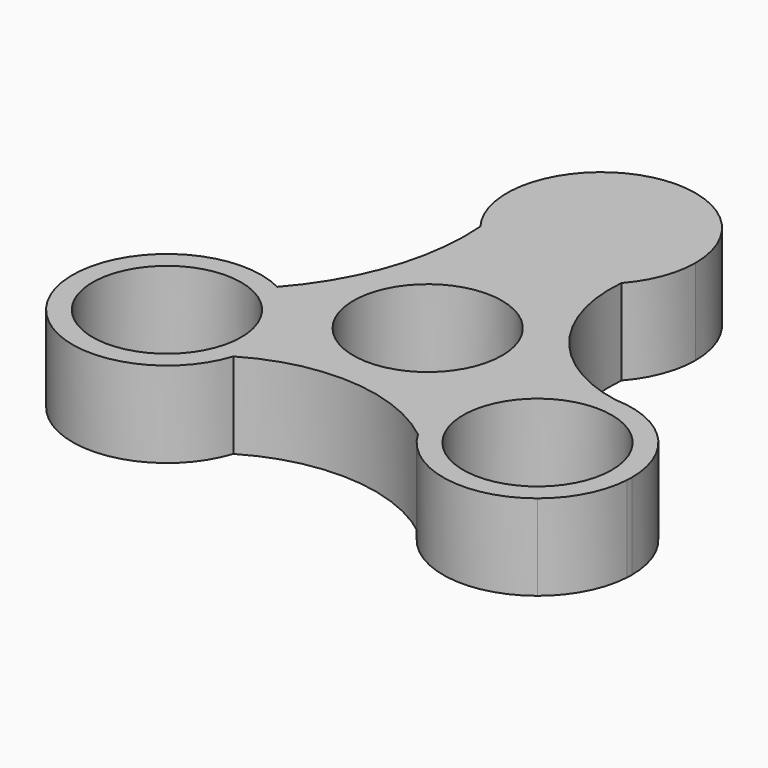
from build123d import *

# Parameters (mm, degrees)
F0_R     = 10.9982
F0_R_2   = 13.97
F1_DEPTH = 12.7


with BuildPart() as f1:
    # F0 (on Top) → F1 (new body)
    with BuildSketch(Plane.XY):
        with BuildLine():
            ThreePointArc((13.97, 32.0970378816), (12.2885629968, 38.7417440057), (7.6490093808, 43.7869290484))
            ThreePointArc((7.6490093808, 43.7869290484), (0, 44.45), (-7.6490093808, 43.7869290484))
            ThreePointArc((-7.6490093808, 43.7869290484), (-13.7655856932, 34.4781196782), (-11.1311920138, 23.6556242351))
            ThreePointArc((-11.1311920138, 23.6556242351), (-0.5487801971, 18.1378208443), (10.4341459432, 22.8078237902))
            ThreePointArc((10.4341459432, 22.8078237902), (13.0561464228, 27.1273356182), (13.97, 32.0970378816))
        make_face()
        with Locations((0, 32.0970378816)):
            Circle(F0_R, mode=Mode.SUBTRACT)
        with BuildLine():
            ThreePointArc((-7.6490093808, 43.7869290484), (0, 44.45), (7.6490093808, 43.7869290484))
            ThreePointArc((7.6490093808, 43.7869290484), (0, 46.0670378816), (-7.6490093808, 43.7869290484))
        make_face()
        with BuildLine():
            ThreePointArc((36.5141532997, -25.3479606439), (40.1954437919, -20.8685438007), (41.7410377882, -15.2803227832))
            ThreePointArc((41.7410377882, -15.2803227832), (39.4500705459, -20.4815632685), (36.5141532997, -25.3479606439))
        make_face()
        with BuildLine():
            ThreePointArc((36.5141532997, -25.3479606439), (39.4500705459, -20.4815632685), (41.7410377882, -15.2803227832))
            ThreePointArc((41.7410377882, -15.2803227832), (41.7603955997, -14.856098108), (41.7668501917, -14.4314810592))
            ThreePointArc((41.7668501917, -14.4314810592), (37.8325982415, -4.7132167552), (28.245782034, -0.4686962295))
            ThreePointArc((28.245782034, -0.4686962295), (15.8040282066, -7.2667674687), (15.7145912135, -21.4443205685))
            ThreePointArc((15.7145912135, -21.4443205685), (25.2199657431, -28.1617602457), (36.5141532997, -25.3479606439))
        make_face()
        with Locations((27.7968501917, -14.4314810592)):
            Circle(F0_R, mode=Mode.SUBTRACT)
        with BuildLine():
            ThreePointArc((-20.0335070466, -2.8032077223), (-36.5219312191, -5.6152601432), (-38.4948294602, -22.2249995463))
            ThreePointArc((-38.4948294602, -22.2249995463), (-24.9413525406, -29.134012338), (-13.1134053752, -19.5668361497))
            ThreePointArc((-13.1134053752, -19.5668361497), (-12.5992608684, -17.4305143709), (-12.4264543073, -15.24))
            ThreePointArc((-12.4264543073, -15.24), (-14.4790033796, -7.9506061031), (-20.0335070466, -2.8032077223))
        make_face()
        with Locations((-26.3964543073, -15.24)):
            Circle(F0_R, mode=Mode.SUBTRACT)
        with BuildLine():
            ThreePointArc((10.4341459432, 22.8078237902), (-0.5487801971, 18.1378208443), (-11.1311920138, 23.6556242351))
            ThreePointArc((-11.1311920138, 23.6556242351), (-12.8966882758, 9.5225930629), (-20.0335070466, -2.8032077223))
            ThreePointArc((-20.0335070466, -2.8032077223), (-14.4790033796, -7.9506061031), (-12.4264543073, -15.24))
            ThreePointArc((-12.4264543073, -15.24), (-12.5992608684, -17.4305143709), (-13.1134053752, -19.5668361497))
            ThreePointArc((-13.1134053752, -19.5668361497), (1.5922377479, -16.0274926586), (15.7145912135, -21.4443205685))
            ThreePointArc((15.7145912135, -21.4443205685), (15.8040282066, -7.2667674687), (28.245782034, -0.4686962295))
            ThreePointArc((28.245782034, -0.4686962295), (14.7899139444, 7.6877788952), (10.4341459432, 22.8078237902))
        make_face()
        Circle(F0_R_2, mode=Mode.SUBTRACT)
        with Locations((0, 32.0970378816)):
            Circle(F0_R)
        Circle(F0_R_2)
        Circle(F0_R, mode=Mode.SUBTRACT)
    extrude(amount=F1_DEPTH)


solid = f1.part
